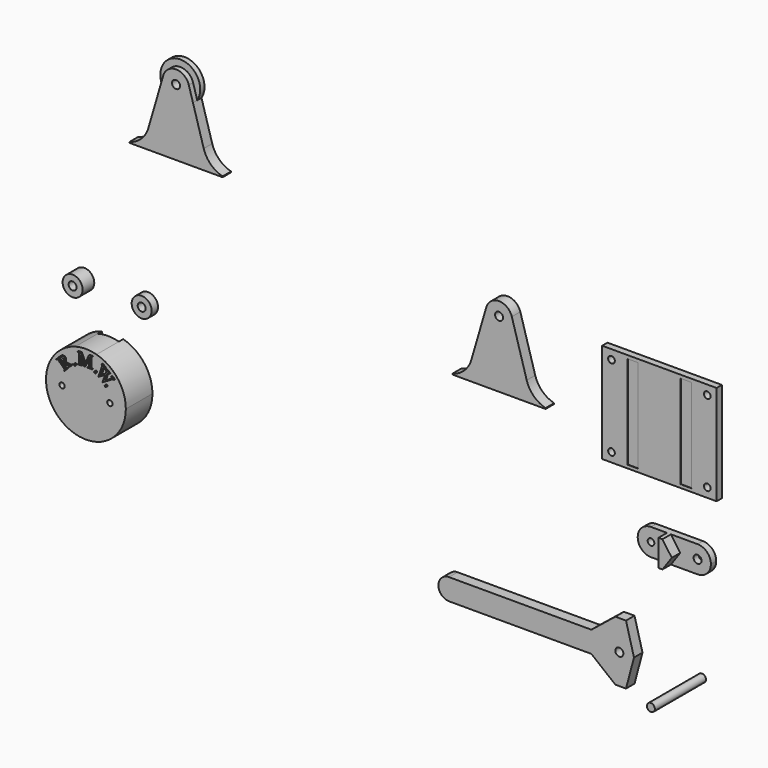
from build123d import *

# Parameters (mm, degrees)
F0_R      = 3
F1_DEPTH  = 8
F2_R      = 3
F3_DEPTH  = 8
F4_R      = 3
F5_DEPTH  = 48
F7_DEPTH  = 21
F6_R      = 2
F8_DEPTH  = 25
F9_DEPTH  = 1
F10_R     = 7.5
F10_R_2   = 3
F12_DEPTH = 6
F11_R     = 7.5
F11_R_2   = 3
F13_DEPTH = 11
F16_DEPTH = 4
F15_R     = 3
F17_DEPTH = 8
F14_W     = 86
F14_H     = 75
F14_R     = 2.5
F14_W_2   = 8
F14_H_2   = 70.1
F18_DEPTH = 5
F19_DEPTH = 4.7
F20_R     = 2.5
F21_DEPTH = 5
F20_R_2   = 7.5
F22_START = 0.2
F20_R_3   = 3
F22_DEPTH = 4.8
F23_DEPTH = 13


# Not quite as in the source:
# - ends of sketch curves that miss each other by under 0.0002 mm in the source are joined


with BuildPart() as f1:
    # F0 (on Front) → F1 (new body)
    with BuildSketch(Plane.XZ):
        with BuildLine():
            Line((91.7526111007, 74.1948067945), (91.7526111007, 73.5597237945))
            Line((91.7526111007, 73.5597237945), (161.7526111007, 73.5597237945))
            Line((161.7526111007, 73.5597237945), (161.7526111007, 74.1948067945))
            ThreePointArc((161.7526111007, 74.1948067945), (152.8321860899, 79.1993001406), (147.5526111007, 87.9597237945))
            Line((147.5526111007, 87.9597237945), (136.3526111007, 126.3597237945))
            ThreePointArc((136.3526111007, 126.3597237945), (126.7526111007, 133.5597237945), (117.1526111007, 126.3597237945))
            Line((117.1526111007, 126.3597237945), (105.9526111007, 87.9597237945))
            ThreePointArc((105.9526111007, 87.9597237945), (100.6730361115, 79.1993001406), (91.7526111007, 74.1948067945))
        make_face()
        with Locations((126.7526111007, 123.5597237945)):
            Circle(F0_R, mode=Mode.SUBTRACT)
    extrude(amount=F1_DEPTH)


with BuildPart() as f3:
    # F2 (on Front) → F3 (new body)
    with BuildSketch(Plane.XZ):
        with BuildLine():
            Line((228.1742408276, -69.2982090712), (222.1742408276, -46.7982090712))
            Line((222.1742408276, -46.7982090712), (214.1742408276, -46.7982090712))
            Line((214.1742408276, -46.7982090712), (196.1742408276, -61.2982090712))
            Line((196.1742408276, -61.2982090712), (89.1742408276, -61.2982090712))
            ThreePointArc((89.1742408276, -61.2982090712), (83.5173865781, -63.6413548217), (81.1742408276, -69.2982090712))
            ThreePointArc((81.1742408276, -69.2982090712), (83.5173865781, -74.9550633207), (89.1742408276, -77.2982090712))
            Line((89.1742408276, -77.2982090712), (196.1742408276, -77.2982090712))
            Line((196.1742408276, -77.2982090712), (214.1742408276, -91.7982090712))
            Line((214.1742408276, -91.7982090712), (222.1742408276, -91.7982090712))
            Line((222.1742408276, -91.7982090712), (228.1742408276, -69.2982090712))
        make_face()
        with Locations((217.1742408276, -69.2982090712)):
            Circle(F2_R, mode=Mode.SUBTRACT)
    extrude(amount=F3_DEPTH)


with BuildPart() as f5:
    # F4 (on Front) → F5 (new body)
    with BuildSketch(Plane.XZ):
        with Locations((272.8815972805, -71.5365037322)):
            Circle(F4_R)
    extrude(amount=F5_DEPTH)


with BuildPart() as f7:
    # F6 (on Front) → F7 (new body)
    with BuildSketch(Plane.XZ):
        with BuildLine():
            Line((-198.1619641029, -16.3318043726), (-198.0776991029, -16.2824186042))
            Line((-198.0776991029, -16.2824186042), (-197.9450911029, -16.2339666042))
            Line((-197.9450911029, -16.2339666042), (-197.8122691029, -16.2133986042))
            Line((-197.8122691029, -16.2133986042), (-197.6792331029, -16.2207146042))
            Line((-197.6792331029, -16.2207146042), (-197.5459821029, -16.2559146042))
            Line((-197.5459821029, -16.2559146042), (-197.4216611029, -16.3151236042))
            Line((-197.4216611029, -16.3151236042), (-197.3154121029, -16.3944676042))
            Line((-197.3154121029, -16.3944676042), (-197.2272371029, -16.4939466042))
            Line((-197.2272371029, -16.4939466042), (-197.1571341029, -16.6135606042))
            Line((-197.1571341029, -16.6135606042), (-197.1097611029, -16.7438786042))
            Line((-197.1097611029, -16.7438786042), (-197.0897731029, -16.8754666042))
            Line((-197.0897731029, -16.8754666042), (-197.0971721029, -17.0083266042))
            Line((-197.0971721029, -17.0083266042), (-197.1319571029, -17.1424586042))
            Line((-197.1319571029, -17.1424586042), (-197.1905861029, -17.2680136042))
            Line((-197.1905861029, -17.2680136042), (-197.2695151029, -17.3751426042))
            Line((-197.2695151029, -17.3751426042), (-197.3687451029, -17.4638476042))
            Line((-197.3687451029, -17.4638476042), (-197.4882761029, -17.5341266042))
            Line((-197.4882761029, -17.5341266042), (-197.6185941029, -17.5814996042))
            Line((-197.6185941029, -17.5814996042), (-197.7501821029, -17.6014866042))
            Line((-197.7501821029, -17.6014866042), (-197.8830431029, -17.5940876042))
            Line((-197.8830431029, -17.5940876042), (-198.0171741029, -17.5593026042))
            Line((-198.0171741029, -17.5593026042), (-198.1427291029, -17.5006746042))
            Line((-198.1427291029, -17.5006746042), (-198.1619641029, -17.4865028638))
            Line((-198.1619641029, -17.4865028638), (-198.1619641029, -63.2965836042))
            ThreePointArc((-198.1619641029, -63.2965836042), (-190.1619641029, -64.3829186042), (-182.1619642084, -63.296583223))
            Line((-182.1619642084, -63.296583223), (-182.1619641029, -17.5489829879))
            Line((-182.1619641029, -17.5489829879), (-182.2444761029, -17.5865666042))
            Line((-182.2444761029, -17.5865666042), (-182.3789311029, -17.6200826042))
            Line((-182.3789311029, -17.6200826042), (-182.5118551029, -17.6262246042))
            Line((-182.5118551029, -17.6262246042), (-182.6432491029, -17.6049946042))
            Line((-182.6432491029, -17.6049946042), (-182.7731131029, -17.5563916042))
            Line((-182.7731131029, -17.5563916042), (-182.8919741029, -17.4849856042))
            Line((-182.8919741029, -17.4849856042), (-182.9903611029, -17.3953476042))
            Line((-182.9903611029, -17.3953476042), (-183.0682741029, -17.2874766042))
            Line((-183.0682741029, -17.2874766042), (-183.1257131029, -17.1613736042))
            Line((-183.1257131029, -17.1613736042), (-183.1592291029, -17.0269186042))
            Line((-183.1592291029, -17.0269186042), (-183.1653711029, -16.8939946042))
            Line((-183.1653711029, -16.8939946042), (-183.1441411029, -16.7626006042))
            Line((-183.1441411029, -16.7626006042), (-183.0955381029, -16.6327366042))
            Line((-183.0955381029, -16.6327366042), (-183.0230321029, -16.5115956042))
            Line((-183.0230321029, -16.5115956042), (-182.9328011029, -16.4119806042))
            Line((-182.9328011029, -16.4119806042), (-182.8248461029, -16.3338916042))
            Line((-182.8248461029, -16.3338916042), (-182.6991651029, -16.2773296042))
            Line((-182.6991651029, -16.2773296042), (-182.5653031029, -16.2450426042))
            Line((-182.5653031029, -16.2450426042), (-182.4328021029, -16.2397766042))
            Line((-182.4328021029, -16.2397766042), (-182.3016621029, -16.2615336042))
            Line((-182.3016621029, -16.2615336042), (-182.1718831029, -16.3103116042))
            Line((-182.1718831029, -16.3103116042), (-182.1619641029, -16.3162483805))
            Line((-182.1619641029, -16.3162483805), (-182.1619641029, -5.4692546042))
            ThreePointArc((-182.1619641029, -5.4692546042), (-190.1619641029, -4.3829186042), (-198.1619642544, -5.4692540565))
            Line((-198.1619642544, -5.4692540565), (-198.1619641029, -16.3318043726))
        make_face()
        Polygon((-190.3483751029, -15.8450716042), (-190.5540121029, -15.8482386042), (-193.9287881029, -8.7884576042), (-193.8418381029, -14.4341396042), (-193.8258881029, -14.7868326042), (-193.7900351029, -15.0659826042), (-193.7646451029, -15.1779796042), (-193.7342781029, -15.2715896042), (-193.6989361029, -15.3468136042), (-193.6586181029, -15.4036526042), (-193.5958461029, -15.4640416042), (-193.5248261029, -15.5161226042), (-193.4455591029, -15.5598956042), (-193.3580441029, -15.5953606042), (-193.2622811029, -15.6225186042), (-193.1582721029, -15.6413676042), (-193.0460141029, -15.6519106042), (-192.9255091029, -15.6541446042), (-192.6264001029, -15.6495376042), (-192.6228491029, -15.8801016042), (-195.5640881029, -15.9253996042), (-195.5676391029, -15.6948366042), (-195.2685301029, -15.6902296042), (-195.1395001029, -15.6831786042), (-195.0203631029, -15.6661506042), (-194.9111181029, -15.6391466042), (-194.8117671029, -15.6021666042), (-194.7223071029, -15.5552106042), (-194.6427401029, -15.4982786042), (-194.5730661029, -15.4313706042), (-194.5132851029, -15.3544866042), (-194.4820451029, -15.2961556042), (-194.4553351029, -15.2219236042), (-194.4331541029, -15.1317886042), (-194.4155041029, -15.0257526042), (-194.3937951029, -14.7659726042), (-194.3902051029, -14.4425856042), (-194.4752351029, -8.9215316042), (-194.4870431029, -8.6607096042), (-194.5138301029, -8.4390746042), (-194.5555951029, -8.2566266042), (-194.6123401029, -8.1133636042), (-194.6664471029, -8.0275206042), (-194.7387451029, -7.9493596042), (-194.8292331029, -7.8788796042), (-194.9379131029, -7.8160816042), (-195.0732921029, -7.7649926042), (-195.2438781029, -7.7296376042), (-195.4496721029, -7.7100176042), (-195.6906731029, -7.7061336042), (-195.6942241029, -7.4755696042), (-193.3013521029, -7.4387176042), (-190.1336601029, -14.0030546042), (-187.2194691029, -7.3450506042), (-184.8265971029, -7.3081976042), (-184.8230461029, -7.5387606042), (-185.1159231029, -7.5432716042), (-185.2464131029, -7.5503456042), (-185.3668161029, -7.5673926042), (-185.4771321029, -7.5944126042), (-185.5773601029, -7.6314056042), (-185.6675011029, -7.6783726042), (-185.7475541029, -7.7353116042), (-185.8175211029, -7.8022246042), (-185.8774001029, -7.8791106042), (-185.9086401029, -7.9374406042), (-185.9353501029, -8.0116736042), (-185.9575301029, -8.1018076042), (-185.9751801029, -8.2078446042), (-185.9968901029, -8.4676236042), (-186.0004801029, -8.7910116042), (-185.9154501029, -14.3120656042), (-185.8991101029, -14.6647526042), (-185.8831851029, -14.8135126042), (-185.8620891029, -14.9438846042), (-185.8358221029, -15.0558676042), (-185.8043851029, -15.1494606042), (-185.7677771029, -15.2246656042), (-185.7259981029, -15.2814826042), (-185.6632261029, -15.3418706042), (-185.5922061029, -15.3939516042), (-185.5129391029, -15.4377246042), (-185.4254241029, -15.4731896042), (-185.3296621029, -15.5003476042), (-185.2256521029, -15.5191976042), (-185.1133941029, -15.5297396042), (-184.9928891029, -15.5319746042), (-184.7000121029, -15.5274636042), (-184.6964611029, -15.7580266042), (-188.2857691029, -15.8133056042), (-188.2893201029, -15.5827426042), (-187.9902111029, -15.5781356042), (-187.8598181029, -15.5710636042), (-187.7397071029, -15.5540206042), (-187.6298781029, -15.5270086042), (-187.5303321029, -15.4900256042), (-187.4410671029, -15.4430726042), (-187.3620851029, -15.3861496042), (-187.2933841029, -15.3192566042), (-187.2349661029, -15.2423926042), (-187.2037261029, -15.1840626042), (-187.1770151029, -15.1098296042), (-187.1548351029, -15.0196956042), (-187.1371851029, -14.9136586042), (-187.1154761029, -14.6538796042), (-187.1118861029, -14.3304916042), (-187.1988351029, -8.6848096042), align=None, mode=Mode.SUBTRACT)
        Polygon((-193.9287881029, -8.7884576042), (-190.5540121029, -15.8482386042), (-190.3483751029, -15.8450716042), (-187.1988351029, -8.6848096042), (-187.1118861029, -14.3304916042), (-187.1154761029, -14.6538796042), (-187.1371851029, -14.9136586042), (-187.1548351029, -15.0196956042), (-187.1770151029, -15.1098296042), (-187.2037261029, -15.1840626042), (-187.2349661029, -15.2423926042), (-187.2933841029, -15.3192566042), (-187.3620851029, -15.3861496042), (-187.4410671029, -15.4430726042), (-187.5303321029, -15.4900256042), (-187.6298781029, -15.5270086042), (-187.7397071029, -15.5540206042), (-187.8598181029, -15.5710636042), (-187.9902111029, -15.5781356042), (-188.2893201029, -15.5827426042), (-188.2857691029, -15.8133056042), (-184.6964611029, -15.7580266042), (-184.7000121029, -15.5274636042), (-184.9928891029, -15.5319746042), (-185.1133941029, -15.5297396042), (-185.2256521029, -15.5191976042), (-185.3296621029, -15.5003476042), (-185.4254241029, -15.4731896042), (-185.5129391029, -15.4377246042), (-185.5922061029, -15.3939516042), (-185.6632261029, -15.3418706042), (-185.7259981029, -15.2814826042), (-185.7677771029, -15.2246656042), (-185.8043851029, -15.1494606042), (-185.8358221029, -15.0558676042), (-185.8620891029, -14.9438846042), (-185.8831851029, -14.8135126042), (-185.8991101029, -14.6647526042), (-185.9154501029, -14.3120656042), (-186.0004801029, -8.7910116042), (-185.9968901029, -8.4676236042), (-185.9751801029, -8.2078446042), (-185.9575301029, -8.1018076042), (-185.9353501029, -8.0116736042), (-185.9086401029, -7.9374406042), (-185.8774001029, -7.8791106042), (-185.8175211029, -7.8022246042), (-185.7475541029, -7.7353116042), (-185.6675011029, -7.6783726042), (-185.5773601029, -7.6314056042), (-185.4771321029, -7.5944126042), (-185.3668161029, -7.5673926042), (-185.2464131029, -7.5503456042), (-185.1159231029, -7.5432716042), (-184.8230461029, -7.5387606042), (-184.8265971029, -7.3081976042), (-187.2194691029, -7.3450506042), (-190.1336601029, -14.0030546042), (-193.3013521029, -7.4387176042), (-195.6942241029, -7.4755696042), (-195.6906731029, -7.7061336042), (-195.4496721029, -7.7100176042), (-195.2438781029, -7.7296376042), (-195.0732921029, -7.7649926042), (-194.9379131029, -7.8160816042), (-194.8292331029, -7.8788796042), (-194.7387451029, -7.9493596042), (-194.6664471029, -8.0275206042), (-194.6123401029, -8.1133636042), (-194.5555951029, -8.2566266042), (-194.5138301029, -8.4390746042), (-194.4870431029, -8.6607096042), (-194.4752351029, -8.9215316042), (-194.3902051029, -14.4425856042), (-194.3937951029, -14.7659726042), (-194.4155041029, -15.0257526042), (-194.4331541029, -15.1317886042), (-194.4553351029, -15.2219236042), (-194.4820451029, -15.2961556042), (-194.5132851029, -15.3544866042), (-194.5730661029, -15.4313706042), (-194.6427401029, -15.4982786042), (-194.7223071029, -15.5552106042), (-194.8117671029, -15.6021666042), (-194.9111181029, -15.6391466042), (-195.0203631029, -15.6661506042), (-195.1395001029, -15.6831786042), (-195.2685301029, -15.6902296042), (-195.5676391029, -15.6948366042), (-195.5640881029, -15.9253996042), (-192.6228491029, -15.8801016042), (-192.6264001029, -15.6495376042), (-192.9255091029, -15.6541446042), (-193.0460141029, -15.6519106042), (-193.1582721029, -15.6413676042), (-193.2622811029, -15.6225186042), (-193.3580441029, -15.5953606042), (-193.4455591029, -15.5598956042), (-193.5248261029, -15.5161226042), (-193.5958461029, -15.4640416042), (-193.6586181029, -15.4036526042), (-193.6989361029, -15.3468136042), (-193.7342781029, -15.2715896042), (-193.7646451029, -15.1779796042), (-193.7900351029, -15.0659826042), (-193.8258881029, -14.7868326042), (-193.8418381029, -14.4341396042), align=None)
        Polygon((-182.1619641029, -17.5489829879), (-182.1619641029, -16.3162483805), (-182.1718831029, -16.3103116042), (-182.3016621029, -16.2615336042), (-182.4328021029, -16.2397766042), (-182.5653031029, -16.2450426042), (-182.6991651029, -16.2773296042), (-182.8248461029, -16.3338916042), (-182.9328011029, -16.4119806042), (-183.0230321029, -16.5115956042), (-183.0955381029, -16.6327366042), (-183.1441411029, -16.7626006042), (-183.1653711029, -16.8939946042), (-183.1592291029, -17.0269186042), (-183.1257131029, -17.1613736042), (-183.0682741029, -17.2874766042), (-182.9903611029, -17.3953476042), (-182.8919741029, -17.4849856042), (-182.7731131029, -17.5563916042), (-182.6432491029, -17.6049946042), (-182.5118551029, -17.6262246042), (-182.3789311029, -17.6200826042), (-182.2444761029, -17.5865666042), align=None)
        Polygon((-197.9450911029, -16.2339666042), (-198.0776991029, -16.2824186042), (-198.1619641029, -16.3318043726), (-198.1619641029, -17.4865028638), (-198.1427291029, -17.5006746042), (-198.0171741029, -17.5593026042), (-197.8830431029, -17.5940876042), (-197.7501821029, -17.6014866042), (-197.6185941029, -17.5814996042), (-197.4882761029, -17.5341266042), (-197.3687451029, -17.4638476042), (-197.2695151029, -17.3751426042), (-197.1905861029, -17.2680136042), (-197.1319571029, -17.1424586042), (-197.0971721029, -17.0083266042), (-197.0897731029, -16.8754666042), (-197.1097611029, -16.7438786042), (-197.1571341029, -16.6135606042), (-197.2272371029, -16.4939466042), (-197.3154121029, -16.3944676042), (-197.4216611029, -16.3151236042), (-197.5459821029, -16.2559146042), (-197.6792331029, -16.2207146042), (-197.8122691029, -16.2133986042), align=None)
    extrude(amount=-F7_DEPTH)

    # F6 (on Front) → F8 (join)
    with BuildSketch(Plane.XZ):
        with BuildLine():
            Line((-198.1973131029, -16.3525216042), (-198.1619641029, -16.3318043726))
            Line((-198.1619641029, -16.3318043726), (-198.1619641029, -5.4692546042))
            ThreePointArc((-198.1619641029, -5.4692546042), (-220.1619641029, -34.3829187375), (-198.1619639974, -63.296583223))
            Line((-198.1619639974, -63.296583223), (-198.1619641029, -17.4865028638))
            Line((-198.1619641029, -17.4865028638), (-198.2498591029, -17.4217446042))
            Line((-198.2498591029, -17.4217446042), (-198.3385631029, -17.3225146042))
            Line((-198.3385631029, -17.3225146042), (-198.4088421029, -17.2029836042))
            Line((-198.4088421029, -17.2029836042), (-198.4572941029, -17.0703756042))
            Line((-198.4572941029, -17.0703756042), (-198.4778621029, -16.9375536042))
            Line((-198.4778621029, -16.9375536042), (-198.4705461029, -16.8045176042))
            Line((-198.4705461029, -16.8045176042), (-198.4353461029, -16.6712666042))
            Line((-198.4353461029, -16.6712666042), (-198.3761371029, -16.5469456042))
            Line((-198.3761371029, -16.5469456042), (-198.2967921029, -16.4406966042))
            Line((-198.2967921029, -16.4406966042), (-198.1973131029, -16.3525216042))
        make_face()
        with Locations((-208.1619641029, -34.3829186042)):
            Circle(F6_R, mode=Mode.SUBTRACT)
        Polygon((-200.0576071029, -17.6949796042), (-199.8936781029, -17.8571486042), (-201.4803091029, -19.4610036042), (-206.3010501029, -18.7158246042), (-206.6559751029, -19.0923246042), (-206.7809131029, -19.2141886042), (-206.9234311029, -19.3449606042), (-205.1777981029, -21.0718476042), (-204.9134341029, -21.3180316042), (-204.7956441029, -21.4153806042), (-204.6874491029, -21.4955656042), (-204.5888491029, -21.5585886042), (-204.4998441029, -21.6044496042), (-204.4204351029, -21.6331476042), (-204.3506201029, -21.6446836042), (-204.2606891029, -21.6451616042), (-204.1716461029, -21.6343526042), (-204.0834901029, -21.6122556042), (-203.9962211029, -21.5788706042), (-203.9098401029, -21.5341976042), (-203.8243451029, -21.4782366042), (-203.7397381029, -21.4109886042), (-203.6560181029, -21.3324516042), (-203.4237211029, -21.0976336042), (-203.2597921029, -21.2598026042), (-205.8062921029, -23.8339466042), (-205.9702221029, -23.6717766042), (-205.7466911029, -23.4458196042), (-205.6596901029, -23.3501196042), (-205.5871531029, -23.2535346042), (-205.5290821029, -23.1560626042), (-205.4854751029, -23.0577056042), (-205.4563331029, -22.9584626042), (-205.4416561029, -22.8583326042), (-205.4414441029, -22.7573176042), (-205.4556971029, -22.6554166042), (-205.4743451029, -22.5938216042), (-205.5076391029, -22.5234906042), (-205.6181611029, -22.3566266042), (-205.7872621029, -22.1548226042), (-206.0149441029, -21.9180806042), (-209.8960961029, -18.0786066042), (-210.1604611029, -17.8324226042), (-210.2782511029, -17.7350736042), (-210.3864451029, -17.6548886042), (-210.4850451029, -17.5918646042), (-210.5740501029, -17.5460046042), (-210.6534601029, -17.5173066042), (-210.7232751029, -17.5057706042), (-210.8143011029, -17.5064006042), (-210.9044401029, -17.5183166042), (-210.9936921029, -17.5415216042), (-211.0820561029, -17.5760146042), (-211.1695331029, -17.6217946042), (-211.2561241029, -17.6788636042), (-211.3418261029, -17.7472196042), (-211.4266421029, -17.8268636042), (-211.6501731029, -18.0528206042), (-211.8141031029, -17.8906516042), (-209.6489201029, -15.7019646042), (-209.1979291029, -15.2635246042), (-208.9892111029, -15.0743486042), (-208.7916771029, -14.9052006042), (-208.6053271029, -14.7560826042), (-208.4301621029, -14.6269926042), (-208.2661811029, -14.5179326042), (-208.1133851029, -14.4289016042), (-207.9646351029, -14.3556606042), (-207.8127931029, -14.2939706042), (-207.6578591029, -14.2438326042), (-207.4998331029, -14.2052456042), (-207.3387151029, -14.1782096042), (-207.1745041029, -14.1627256042), (-207.0072021029, -14.1587926042), (-206.8368071029, -14.1664106042), (-206.6675141029, -14.1869806042), (-206.5035131029, -14.2219016042), (-206.3448061029, -14.2711726042), (-206.1913921029, -14.3347956042), (-206.0432721029, -14.4127686042), (-205.9004451029, -14.5050926042), (-205.7629121029, -14.6117676042), (-205.6306721029, -14.7327946042), (-205.5000841029, -14.8731436042), (-205.3852271029, -15.0202576042), (-205.2861021029, -15.1741356042), (-205.2027091029, -15.3347766042), (-205.1350481029, -15.5021826042), (-205.0831191029, -15.6763536042), (-205.0469221029, -15.8572876042), (-205.0264561029, -16.0449856042), (-205.0237241029, -16.2385636042), (-205.0407281029, -16.4371366042), (-205.0774661029, -16.6407056042), (-205.1339391029, -16.8492706042), (-205.2101481029, -17.0628296042), (-205.3060911029, -17.2813856042), (-205.4217701029, -17.5049356042), (-205.5571841029, -17.7334816042), (-202.6064751029, -18.1979026042), (-202.1315651029, -18.2617176042), (-201.7212911029, -18.2911766042), (-201.5403921029, -18.2930236042), (-201.3756531029, -18.2862816042), (-201.2270721029, -18.2709506042), (-201.0946511029, -18.2470306042), (-200.9696481029, -18.2137176042), (-200.8433221029, -18.1702056042), (-200.7156751029, -18.1164966042), (-200.5867061029, -18.0525896042), (-200.4564141029, -17.9784836042), (-200.3248011029, -17.8941806042), align=None, mode=Mode.SUBTRACT)
        with BuildLine():
            ThreePointArc((-160.1619641029, -34.3829186042), (-166.2872912827, -16.2170165422), (-182.1619639514, -5.4692540565))
            Line((-182.1619639514, -5.4692540565), (-182.1619641029, -16.3162483805))
            Line((-182.1619641029, -16.3162483805), (-182.0507421029, -16.3828176042))
            Line((-182.0507421029, -16.3828176042), (-181.9511271029, -16.4730486042))
            Line((-181.9511271029, -16.4730486042), (-181.8730381029, -16.5810036042))
            Line((-181.8730381029, -16.5810036042), (-181.8164761029, -16.7066846042))
            Line((-181.8164761029, -16.7066846042), (-181.7841891029, -16.8405466042))
            Line((-181.7841891029, -16.8405466042), (-181.7789231029, -16.9730476042))
            Line((-181.7789231029, -16.9730476042), (-181.8006801029, -17.1041876042))
            Line((-181.8006801029, -17.1041876042), (-181.8494581029, -17.2339666042))
            Line((-181.8494581029, -17.2339666042), (-181.9208641029, -17.3528276042))
            Line((-181.9208641029, -17.3528276042), (-182.0105021029, -17.4512146042))
            Line((-182.0105021029, -17.4512146042), (-182.1183731029, -17.5291276042))
            Line((-182.1183731029, -17.5291276042), (-182.1619641029, -17.5489829879))
            Line((-182.1619641029, -17.5489829879), (-182.1619641029, -63.2965836042))
            ThreePointArc((-182.1619641029, -63.2965836042), (-166.2872913634, -52.5488207723), (-160.1619641029, -34.3829186042))
        make_face()
        with Locations((-172.1619641029, -34.3829186042)):
            Circle(F6_R, mode=Mode.SUBTRACT)
        Polygon((-174.0892951029, -22.9184336042), (-173.9963871029, -23.0213406042), (-173.9220431029, -23.1413636042), (-173.8749611029, -23.2672526042), (-173.8551391029, -23.3990076042), (-173.8625781029, -23.5366276042), (-173.8953381029, -23.6703746042), (-173.9514811029, -23.7905096042), (-174.0310061029, -23.8970306042), (-174.1339141029, -23.9899386042), (-174.2519131029, -24.0627616042), (-174.3767111029, -24.1090246042), (-174.5083101029, -24.1287296042), (-174.6467101029, -24.1218756042), (-174.7815471029, -24.0899346042), (-174.9024591029, -24.0343766042), (-175.0094481029, -23.9552016042), (-175.1025121029, -23.8524116042), (-175.1753341029, -23.7344126042), (-175.2215981029, -23.6096146042), (-175.2413031029, -23.4780156042), (-175.2344491029, -23.3396156042), (-175.2025071029, -23.2047786042), (-175.1469491029, -23.0838656042), (-175.0677751029, -22.9768776042), (-174.9649851029, -22.8838136042), (-174.8449621029, -22.8094706042), (-174.7190731029, -22.7623876042), (-174.5873181029, -22.7425656042), (-174.4496981029, -22.7500046042), (-174.3159501029, -22.7827656042), (-174.1958161029, -22.8389086042), align=None, mode=Mode.SUBTRACT)
        Polygon((-170.2892841029, -15.7694166042), (-168.3366211029, -17.3687426042), (-168.4827321029, -17.5471346042), (-168.6091621029, -17.4531486042), (-168.7329161029, -17.3804856042), (-168.8539961029, -17.3291466042), (-168.9724021029, -17.2991306042), (-169.0967101029, -17.2904606042), (-169.2355011029, -17.3031596042), (-169.3887721029, -17.3372276042), (-169.5565251029, -17.3926656042), (-169.7047171029, -17.4611036042), (-169.9146511029, -17.5766476042), (-170.1863281029, -17.7392976042), (-170.5197481029, -17.9490536042), (-176.6584381029, -21.7261286042), (-176.8512931029, -21.5681706042), (-174.9173611029, -16.1677986042), (-179.8212701029, -19.1356156042), (-179.9948401029, -18.9934526042), (-177.4913391029, -11.9731406042), (-177.2726431029, -11.3446726042), (-177.1777641029, -11.0296636042), (-177.1601301029, -10.9008646042), (-177.1608611029, -10.7766606042), (-177.1799551029, -10.6570516042), (-177.2174141029, -10.5420366042), (-177.2760041029, -10.4288476042), (-177.3584911029, -10.3147136042), (-177.4648761029, -10.1996356042), (-177.5951591029, -10.0836136042), (-177.4490471029, -9.9052226042), (-175.0287101029, -11.8875966042), (-175.1748211029, -12.0659886042), (-175.2905341029, -11.9712136042), (-175.4166911029, -11.8799686042), (-175.5396281029, -11.8155276042), (-175.6593451029, -11.7778926042), (-175.7758421029, -11.7670616042), (-175.8847591029, -11.7795566042), (-175.9817381029, -11.8119006042), (-176.0667781029, -11.8640916042), (-176.1398801029, -11.9361316042), (-176.2181871029, -12.0587866042), (-176.3148971029, -12.2580056042), (-176.4300081029, -12.5337856042), (-176.5635201029, -12.8861286042), (-178.2813621029, -17.6095766042), (-174.6415771029, -15.3786516042), (-174.3842521029, -14.6710556042), (-174.1791821029, -14.1059426042), (-174.1355511029, -13.9463256042), (-174.1008571029, -13.7914736042), (-174.0751001029, -13.6413846042), (-174.0582791029, -13.4960596042), (-174.0590831029, -13.3544256042), (-174.0861971029, -13.2154086042), (-174.1455231029, -13.0419536042), (-174.2245941029, -12.8926046042), (-174.2666611029, -12.8370036042), (-174.3249481029, -12.7741596042), (-174.4901841029, -12.6267396042), (-174.3440721029, -12.4483476042), (-171.7983791029, -14.5333946042), (-171.9444901029, -14.7117866042), (-172.1180601029, -14.5696236042), (-172.2499421029, -14.4736896042), (-172.3755911029, -14.4070286042), (-172.4950071029, -14.3696396042), (-172.6081891029, -14.3615236042), (-172.7146151029, -14.3795836042), (-172.8137641029, -14.4207226042), (-172.9056341029, -14.4849416042), (-172.9902271029, -14.5722406042), (-173.0961221029, -14.7291946042), (-173.2124131029, -14.9541636042), (-173.3390981029, -15.2471496042), (-173.4761781029, -15.6081506042), (-175.1329941029, -20.1882426042), (-170.9392081029, -17.6054946042), (-170.6203191029, -17.4054876042), (-170.3654631029, -17.2295636042), (-170.1746391029, -17.0777246042), (-170.0478471029, -16.9499696042), (-170.0075441029, -16.8918486042), (-169.9774611029, -16.8283786042), (-169.9575971029, -16.7595586042), (-169.9479531029, -16.6853896042), (-169.9486401029, -16.6103106042), (-169.9597711029, -16.5387626042), (-169.9813451029, -16.4707436042), (-170.0133631029, -16.4062546042), (-170.0877131029, -16.2960166042), (-170.1828341029, -16.1828626042), (-170.2987291029, -16.0667936042), (-170.4353951029, -15.9478086042), align=None, mode=Mode.SUBTRACT)
        Polygon((-201.4803091029, -19.4610036042), (-199.8936781029, -17.8571486042), (-200.0576071029, -17.6949796042), (-200.3248011029, -17.8941806042), (-200.4564141029, -17.9784836042), (-200.5867061029, -18.0525896042), (-200.7156751029, -18.1164966042), (-200.8433221029, -18.1702056042), (-200.9696481029, -18.2137176042), (-201.0946511029, -18.2470306042), (-201.2270721029, -18.2709506042), (-201.3756531029, -18.2862816042), (-201.5403921029, -18.2930236042), (-201.7212911029, -18.2911766042), (-202.1315651029, -18.2617176042), (-202.6064751029, -18.1979026042), (-205.5571841029, -17.7334816042), (-205.4217701029, -17.5049356042), (-205.3060911029, -17.2813856042), (-205.2101481029, -17.0628296042), (-205.1339391029, -16.8492706042), (-205.0774661029, -16.6407056042), (-205.0407281029, -16.4371366042), (-205.0237241029, -16.2385636042), (-205.0264561029, -16.0449856042), (-205.0469221029, -15.8572876042), (-205.0831191029, -15.6763536042), (-205.1350481029, -15.5021826042), (-205.2027091029, -15.3347766042), (-205.2861021029, -15.1741356042), (-205.3852271029, -15.0202576042), (-205.5000841029, -14.8731436042), (-205.6306721029, -14.7327946042), (-205.7629121029, -14.6117676042), (-205.9004451029, -14.5050926042), (-206.0432721029, -14.4127686042), (-206.1913921029, -14.3347956042), (-206.3448061029, -14.2711726042), (-206.5035131029, -14.2219016042), (-206.6675141029, -14.1869806042), (-206.8368071029, -14.1664106042), (-207.0072021029, -14.1587926042), (-207.1745041029, -14.1627256042), (-207.3387151029, -14.1782096042), (-207.4998331029, -14.2052456042), (-207.6578591029, -14.2438326042), (-207.8127931029, -14.2939706042), (-207.9646351029, -14.3556606042), (-208.1133851029, -14.4289016042), (-208.2661811029, -14.5179326042), (-208.4301621029, -14.6269926042), (-208.6053271029, -14.7560826042), (-208.7916771029, -14.9052006042), (-208.9892111029, -15.0743486042), (-209.1979291029, -15.2635246042), (-209.6489201029, -15.7019646042), (-211.8141031029, -17.8906516042), (-211.6501731029, -18.0528206042), (-211.4266421029, -17.8268636042), (-211.3418261029, -17.7472196042), (-211.2561241029, -17.6788636042), (-211.1695331029, -17.6217946042), (-211.0820561029, -17.5760146042), (-210.9936921029, -17.5415216042), (-210.9044401029, -17.5183166042), (-210.8143011029, -17.5064006042), (-210.7232751029, -17.5057706042), (-210.6534601029, -17.5173066042), (-210.5740501029, -17.5460046042), (-210.4850451029, -17.5918646042), (-210.3864451029, -17.6548886042), (-210.2782511029, -17.7350736042), (-210.1604611029, -17.8324226042), (-209.8960961029, -18.0786066042), (-206.0149441029, -21.9180806042), (-205.7872621029, -22.1548226042), (-205.6181611029, -22.3566266042), (-205.5076391029, -22.5234906042), (-205.4743451029, -22.5938216042), (-205.4556971029, -22.6554166042), (-205.4414441029, -22.7573176042), (-205.4416561029, -22.8583326042), (-205.4563331029, -22.9584626042), (-205.4854751029, -23.0577056042), (-205.5290821029, -23.1560626042), (-205.5871531029, -23.2535346042), (-205.6596901029, -23.3501196042), (-205.7466911029, -23.4458196042), (-205.9702221029, -23.6717766042), (-205.8062921029, -23.8339466042), (-203.2597921029, -21.2598026042), (-203.4237211029, -21.0976336042), (-203.6560181029, -21.3324516042), (-203.7397381029, -21.4109886042), (-203.8243451029, -21.4782366042), (-203.9098401029, -21.5341976042), (-203.9962211029, -21.5788706042), (-204.0834901029, -21.6122556042), (-204.1716461029, -21.6343526042), (-204.2606891029, -21.6451616042), (-204.3506201029, -21.6446836042), (-204.4204351029, -21.6331476042), (-204.4998441029, -21.6044496042), (-204.5888491029, -21.5585886042), (-204.6874491029, -21.4955656042), (-204.7956441029, -21.4153806042), (-204.9134341029, -21.3180316042), (-205.1777981029, -21.0718476042), (-206.9234311029, -19.3449606042), (-206.7809131029, -19.2141886042), (-206.6559751029, -19.0923246042), (-206.3010501029, -18.7158246042), align=None)
        Polygon((-207.0557021029, -18.9248176042), (-207.2025551029, -19.0688346042), (-209.7013791029, -16.5968446042), (-209.5324821029, -16.3524526042), (-209.3755261029, -16.1411766042), (-209.2305101029, -15.9630176042), (-209.0974341029, -15.8179736042), (-208.9519161029, -15.6818826042), (-208.8024441029, -15.5638116042), (-208.6490181029, -15.4637596042), (-208.4916401029, -15.3817276042), (-208.3303081029, -15.3177146042), (-208.1650231029, -15.2717206042), (-207.9957851029, -15.2437456042), (-207.8225931029, -15.2337906042), (-207.6495811029, -15.2416016042), (-207.4808811029, -15.2669256042), (-207.3164941029, -15.3097626042), (-207.1564181029, -15.3701126042), (-207.0006561029, -15.4479756042), (-206.8492051029, -15.5433516042), (-206.7020671029, -15.6562416042), (-206.5592411029, -15.7866436042), (-206.4251791029, -15.9327586042), (-206.3109771029, -16.0862106042), (-206.2166351029, -16.2470006042), (-206.1421531029, -16.4151266042), (-206.0875311029, -16.5905906042), (-206.0527701029, -16.7733916042), (-206.0378691029, -16.9635296042), (-206.0428281029, -17.1610056042), (-206.0700721029, -17.3630086042), (-206.1220271029, -17.5667286042), (-206.1986921029, -17.7721656042), (-206.3000681029, -17.9793196042), (-206.4261551029, -18.1881906042), (-206.5769521029, -18.3987786042), (-206.7524601029, -18.6110846042), (-206.9526781029, -18.8251066042), align=None, mode=Mode.SUBTRACT)
        Polygon((-209.7013791029, -16.5968446042), (-207.2025551029, -19.0688346042), (-207.0557021029, -18.9248176042), (-206.9526781029, -18.8251066042), (-206.7524601029, -18.6110846042), (-206.5769521029, -18.3987786042), (-206.4261551029, -18.1881906042), (-206.3000681029, -17.9793196042), (-206.1986921029, -17.7721656042), (-206.1220271029, -17.5667286042), (-206.0700721029, -17.3630086042), (-206.0428281029, -17.1610056042), (-206.0378691029, -16.9635296042), (-206.0527701029, -16.7733916042), (-206.0875311029, -16.5905906042), (-206.1421531029, -16.4151266042), (-206.2166351029, -16.2470006042), (-206.3109771029, -16.0862106042), (-206.4251791029, -15.9327586042), (-206.5592411029, -15.7866436042), (-206.7020671029, -15.6562416042), (-206.8492051029, -15.5433516042), (-207.0006561029, -15.4479756042), (-207.1564181029, -15.3701126042), (-207.3164941029, -15.3097626042), (-207.4808811029, -15.2669256042), (-207.6495811029, -15.2416016042), (-207.8225931029, -15.2337906042), (-207.9957851029, -15.2437456042), (-208.1650231029, -15.2717206042), (-208.3303081029, -15.3177146042), (-208.4916401029, -15.3817276042), (-208.6490181029, -15.4637596042), (-208.8024441029, -15.5638116042), (-208.9519161029, -15.6818826042), (-209.0974341029, -15.8179736042), (-209.2305101029, -15.9630176042), (-209.3755261029, -16.1411766042), (-209.5324821029, -16.3524526042), align=None)
        Polygon((-198.1619641029, -17.4865028638), (-198.1619641029, -16.3318043726), (-198.1973131029, -16.3525216042), (-198.2967921029, -16.4406966042), (-198.3761371029, -16.5469456042), (-198.4353461029, -16.6712666042), (-198.4705461029, -16.8045176042), (-198.4778621029, -16.9375536042), (-198.4572941029, -17.0703756042), (-198.4088421029, -17.2029836042), (-198.3385631029, -17.3225146042), (-198.2498591029, -17.4217446042), align=None)
        Polygon((-182.0507421029, -16.3828176042), (-182.1619641029, -16.3162483805), (-182.1619641029, -17.5489829879), (-182.1183731029, -17.5291276042), (-182.0105021029, -17.4512146042), (-181.9208641029, -17.3528276042), (-181.8494581029, -17.2339666042), (-181.8006801029, -17.1041876042), (-181.7789231029, -16.9730476042), (-181.7841891029, -16.8405466042), (-181.8164761029, -16.7066846042), (-181.8730381029, -16.5810036042), (-181.9511271029, -16.4730486042), align=None)
        Polygon((-168.4827321029, -17.5471346042), (-168.3366211029, -17.3687426042), (-170.2892841029, -15.7694166042), (-170.4353951029, -15.9478086042), (-170.2987291029, -16.0667936042), (-170.1828341029, -16.1828626042), (-170.0877131029, -16.2960166042), (-170.0133631029, -16.4062546042), (-169.9813451029, -16.4707436042), (-169.9597711029, -16.5387626042), (-169.9486401029, -16.6103106042), (-169.9479531029, -16.6853896042), (-169.9575971029, -16.7595586042), (-169.9774611029, -16.8283786042), (-170.0075441029, -16.8918486042), (-170.0478471029, -16.9499696042), (-170.1746391029, -17.0777246042), (-170.3654631029, -17.2295636042), (-170.6203191029, -17.4054876042), (-170.9392081029, -17.6054946042), (-175.1329941029, -20.1882426042), (-173.4761781029, -15.6081506042), (-173.3390981029, -15.2471496042), (-173.2124131029, -14.9541636042), (-173.0961221029, -14.7291946042), (-172.9902271029, -14.5722406042), (-172.9056341029, -14.4849416042), (-172.8137641029, -14.4207226042), (-172.7146151029, -14.3795836042), (-172.6081891029, -14.3615236042), (-172.4950071029, -14.3696396042), (-172.3755911029, -14.4070286042), (-172.2499421029, -14.4736896042), (-172.1180601029, -14.5696236042), (-171.9444901029, -14.7117866042), (-171.7983791029, -14.5333946042), (-174.3440721029, -12.4483476042), (-174.4901841029, -12.6267396042), (-174.3249481029, -12.7741596042), (-174.2666611029, -12.8370036042), (-174.2245941029, -12.8926046042), (-174.1455231029, -13.0419536042), (-174.0861971029, -13.2154086042), (-174.0590831029, -13.3544256042), (-174.0582791029, -13.4960596042), (-174.0751001029, -13.6413846042), (-174.1008571029, -13.7914736042), (-174.1355511029, -13.9463256042), (-174.1791821029, -14.1059426042), (-174.3842521029, -14.6710556042), (-174.6415771029, -15.3786516042), (-178.2813621029, -17.6095766042), (-176.5635201029, -12.8861286042), (-176.4300081029, -12.5337856042), (-176.3148971029, -12.2580056042), (-176.2181871029, -12.0587866042), (-176.1398801029, -11.9361316042), (-176.0667781029, -11.8640916042), (-175.9817381029, -11.8119006042), (-175.8847591029, -11.7795566042), (-175.7758421029, -11.7670616042), (-175.6593451029, -11.7778926042), (-175.5396281029, -11.8155276042), (-175.4166911029, -11.8799686042), (-175.2905341029, -11.9712136042), (-175.1748211029, -12.0659886042), (-175.0287101029, -11.8875966042), (-177.4490471029, -9.9052226042), (-177.5951591029, -10.0836136042), (-177.4648761029, -10.1996356042), (-177.3584911029, -10.3147136042), (-177.2760041029, -10.4288476042), (-177.2174141029, -10.5420366042), (-177.1799551029, -10.6570516042), (-177.1608611029, -10.7766606042), (-177.1601301029, -10.9008646042), (-177.1777641029, -11.0296636042), (-177.2726431029, -11.3446726042), (-177.4913391029, -11.9731406042), (-179.9948401029, -18.9934526042), (-179.8212701029, -19.1356156042), (-174.9173611029, -16.1677986042), (-176.8512931029, -21.5681706042), (-176.6584381029, -21.7261286042), (-170.5197481029, -17.9490536042), (-170.1863281029, -17.7392976042), (-169.9146511029, -17.5766476042), (-169.7047171029, -17.4611036042), (-169.5565251029, -17.3926656042), (-169.3887721029, -17.3372276042), (-169.2355011029, -17.3031596042), (-169.0967101029, -17.2904606042), (-168.9724021029, -17.2991306042), (-168.8539961029, -17.3291466042), (-168.7329161029, -17.3804856042), (-168.6091621029, -17.4531486042), align=None)
        Polygon((-173.9220431029, -23.1413636042), (-173.9963871029, -23.0213406042), (-174.0892951029, -22.9184336042), (-174.1958161029, -22.8389086042), (-174.3159501029, -22.7827656042), (-174.4496981029, -22.7500046042), (-174.5873181029, -22.7425656042), (-174.7190731029, -22.7623876042), (-174.8449621029, -22.8094706042), (-174.9649851029, -22.8838136042), (-175.0677751029, -22.9768776042), (-175.1469491029, -23.0838656042), (-175.2025071029, -23.2047786042), (-175.2344491029, -23.3396156042), (-175.2413031029, -23.4780156042), (-175.2215981029, -23.6096146042), (-175.1753341029, -23.7344126042), (-175.1025121029, -23.8524116042), (-175.0094481029, -23.9552016042), (-174.9024591029, -24.0343766042), (-174.7815471029, -24.0899346042), (-174.6467101029, -24.1218756042), (-174.5083101029, -24.1287296042), (-174.3767111029, -24.1090246042), (-174.2519131029, -24.0627616042), (-174.1339141029, -23.9899386042), (-174.0310061029, -23.8970306042), (-173.9514811029, -23.7905096042), (-173.8953381029, -23.6703746042), (-173.8625781029, -23.5366276042), (-173.8551391029, -23.3990076042), (-173.8749611029, -23.2672526042), align=None)
    extrude(amount=-F8_DEPTH)

    # F6 (on Front) → F9 (join)
    with BuildSketch(Plane.XZ):
        Polygon((-201.4803091029, -19.4610036042), (-199.8936781029, -17.8571486042), (-200.0576071029, -17.6949796042), (-200.3248011029, -17.8941806042), (-200.4564141029, -17.9784836042), (-200.5867061029, -18.0525896042), (-200.7156751029, -18.1164966042), (-200.8433221029, -18.1702056042), (-200.9696481029, -18.2137176042), (-201.0946511029, -18.2470306042), (-201.2270721029, -18.2709506042), (-201.3756531029, -18.2862816042), (-201.5403921029, -18.2930236042), (-201.7212911029, -18.2911766042), (-202.1315651029, -18.2617176042), (-202.6064751029, -18.1979026042), (-205.5571841029, -17.7334816042), (-205.4217701029, -17.5049356042), (-205.3060911029, -17.2813856042), (-205.2101481029, -17.0628296042), (-205.1339391029, -16.8492706042), (-205.0774661029, -16.6407056042), (-205.0407281029, -16.4371366042), (-205.0237241029, -16.2385636042), (-205.0264561029, -16.0449856042), (-205.0469221029, -15.8572876042), (-205.0831191029, -15.6763536042), (-205.1350481029, -15.5021826042), (-205.2027091029, -15.3347766042), (-205.2861021029, -15.1741356042), (-205.3852271029, -15.0202576042), (-205.5000841029, -14.8731436042), (-205.6306721029, -14.7327946042), (-205.7629121029, -14.6117676042), (-205.9004451029, -14.5050926042), (-206.0432721029, -14.4127686042), (-206.1913921029, -14.3347956042), (-206.3448061029, -14.2711726042), (-206.5035131029, -14.2219016042), (-206.6675141029, -14.1869806042), (-206.8368071029, -14.1664106042), (-207.0072021029, -14.1587926042), (-207.1745041029, -14.1627256042), (-207.3387151029, -14.1782096042), (-207.4998331029, -14.2052456042), (-207.6578591029, -14.2438326042), (-207.8127931029, -14.2939706042), (-207.9646351029, -14.3556606042), (-208.1133851029, -14.4289016042), (-208.2661811029, -14.5179326042), (-208.4301621029, -14.6269926042), (-208.6053271029, -14.7560826042), (-208.7916771029, -14.9052006042), (-208.9892111029, -15.0743486042), (-209.1979291029, -15.2635246042), (-209.6489201029, -15.7019646042), (-211.8141031029, -17.8906516042), (-211.6501731029, -18.0528206042), (-211.4266421029, -17.8268636042), (-211.3418261029, -17.7472196042), (-211.2561241029, -17.6788636042), (-211.1695331029, -17.6217946042), (-211.0820561029, -17.5760146042), (-210.9936921029, -17.5415216042), (-210.9044401029, -17.5183166042), (-210.8143011029, -17.5064006042), (-210.7232751029, -17.5057706042), (-210.6534601029, -17.5173066042), (-210.5740501029, -17.5460046042), (-210.4850451029, -17.5918646042), (-210.3864451029, -17.6548886042), (-210.2782511029, -17.7350736042), (-210.1604611029, -17.8324226042), (-209.8960961029, -18.0786066042), (-206.0149441029, -21.9180806042), (-205.7872621029, -22.1548226042), (-205.6181611029, -22.3566266042), (-205.5076391029, -22.5234906042), (-205.4743451029, -22.5938216042), (-205.4556971029, -22.6554166042), (-205.4414441029, -22.7573176042), (-205.4416561029, -22.8583326042), (-205.4563331029, -22.9584626042), (-205.4854751029, -23.0577056042), (-205.5290821029, -23.1560626042), (-205.5871531029, -23.2535346042), (-205.6596901029, -23.3501196042), (-205.7466911029, -23.4458196042), (-205.9702221029, -23.6717766042), (-205.8062921029, -23.8339466042), (-203.2597921029, -21.2598026042), (-203.4237211029, -21.0976336042), (-203.6560181029, -21.3324516042), (-203.7397381029, -21.4109886042), (-203.8243451029, -21.4782366042), (-203.9098401029, -21.5341976042), (-203.9962211029, -21.5788706042), (-204.0834901029, -21.6122556042), (-204.1716461029, -21.6343526042), (-204.2606891029, -21.6451616042), (-204.3506201029, -21.6446836042), (-204.4204351029, -21.6331476042), (-204.4998441029, -21.6044496042), (-204.5888491029, -21.5585886042), (-204.6874491029, -21.4955656042), (-204.7956441029, -21.4153806042), (-204.9134341029, -21.3180316042), (-205.1777981029, -21.0718476042), (-206.9234311029, -19.3449606042), (-206.7809131029, -19.2141886042), (-206.6559751029, -19.0923246042), (-206.3010501029, -18.7158246042), align=None)
        Polygon((-207.0557021029, -18.9248176042), (-207.2025551029, -19.0688346042), (-209.7013791029, -16.5968446042), (-209.5324821029, -16.3524526042), (-209.3755261029, -16.1411766042), (-209.2305101029, -15.9630176042), (-209.0974341029, -15.8179736042), (-208.9519161029, -15.6818826042), (-208.8024441029, -15.5638116042), (-208.6490181029, -15.4637596042), (-208.4916401029, -15.3817276042), (-208.3303081029, -15.3177146042), (-208.1650231029, -15.2717206042), (-207.9957851029, -15.2437456042), (-207.8225931029, -15.2337906042), (-207.6495811029, -15.2416016042), (-207.4808811029, -15.2669256042), (-207.3164941029, -15.3097626042), (-207.1564181029, -15.3701126042), (-207.0006561029, -15.4479756042), (-206.8492051029, -15.5433516042), (-206.7020671029, -15.6562416042), (-206.5592411029, -15.7866436042), (-206.4251791029, -15.9327586042), (-206.3109771029, -16.0862106042), (-206.2166351029, -16.2470006042), (-206.1421531029, -16.4151266042), (-206.0875311029, -16.5905906042), (-206.0527701029, -16.7733916042), (-206.0378691029, -16.9635296042), (-206.0428281029, -17.1610056042), (-206.0700721029, -17.3630086042), (-206.1220271029, -17.5667286042), (-206.1986921029, -17.7721656042), (-206.3000681029, -17.9793196042), (-206.4261551029, -18.1881906042), (-206.5769521029, -18.3987786042), (-206.7524601029, -18.6110846042), (-206.9526781029, -18.8251066042), align=None, mode=Mode.SUBTRACT)
        Polygon((-197.9450911029, -16.2339666042), (-198.0776991029, -16.2824186042), (-198.1619641029, -16.3318043726), (-198.1619641029, -17.4865028638), (-198.1427291029, -17.5006746042), (-198.0171741029, -17.5593026042), (-197.8830431029, -17.5940876042), (-197.7501821029, -17.6014866042), (-197.6185941029, -17.5814996042), (-197.4882761029, -17.5341266042), (-197.3687451029, -17.4638476042), (-197.2695151029, -17.3751426042), (-197.1905861029, -17.2680136042), (-197.1319571029, -17.1424586042), (-197.0971721029, -17.0083266042), (-197.0897731029, -16.8754666042), (-197.1097611029, -16.7438786042), (-197.1571341029, -16.6135606042), (-197.2272371029, -16.4939466042), (-197.3154121029, -16.3944676042), (-197.4216611029, -16.3151236042), (-197.5459821029, -16.2559146042), (-197.6792331029, -16.2207146042), (-197.8122691029, -16.2133986042), align=None)
        Polygon((-198.1619641029, -17.4865028638), (-198.1619641029, -16.3318043726), (-198.1973131029, -16.3525216042), (-198.2967921029, -16.4406966042), (-198.3761371029, -16.5469456042), (-198.4353461029, -16.6712666042), (-198.4705461029, -16.8045176042), (-198.4778621029, -16.9375536042), (-198.4572941029, -17.0703756042), (-198.4088421029, -17.2029836042), (-198.3385631029, -17.3225146042), (-198.2498591029, -17.4217446042), align=None)
        Polygon((-193.9287881029, -8.7884576042), (-190.5540121029, -15.8482386042), (-190.3483751029, -15.8450716042), (-187.1988351029, -8.6848096042), (-187.1118861029, -14.3304916042), (-187.1154761029, -14.6538796042), (-187.1371851029, -14.9136586042), (-187.1548351029, -15.0196956042), (-187.1770151029, -15.1098296042), (-187.2037261029, -15.1840626042), (-187.2349661029, -15.2423926042), (-187.2933841029, -15.3192566042), (-187.3620851029, -15.3861496042), (-187.4410671029, -15.4430726042), (-187.5303321029, -15.4900256042), (-187.6298781029, -15.5270086042), (-187.7397071029, -15.5540206042), (-187.8598181029, -15.5710636042), (-187.9902111029, -15.5781356042), (-188.2893201029, -15.5827426042), (-188.2857691029, -15.8133056042), (-184.6964611029, -15.7580266042), (-184.7000121029, -15.5274636042), (-184.9928891029, -15.5319746042), (-185.1133941029, -15.5297396042), (-185.2256521029, -15.5191976042), (-185.3296621029, -15.5003476042), (-185.4254241029, -15.4731896042), (-185.5129391029, -15.4377246042), (-185.5922061029, -15.3939516042), (-185.6632261029, -15.3418706042), (-185.7259981029, -15.2814826042), (-185.7677771029, -15.2246656042), (-185.8043851029, -15.1494606042), (-185.8358221029, -15.0558676042), (-185.8620891029, -14.9438846042), (-185.8831851029, -14.8135126042), (-185.8991101029, -14.6647526042), (-185.9154501029, -14.3120656042), (-186.0004801029, -8.7910116042), (-185.9968901029, -8.4676236042), (-185.9751801029, -8.2078446042), (-185.9575301029, -8.1018076042), (-185.9353501029, -8.0116736042), (-185.9086401029, -7.9374406042), (-185.8774001029, -7.8791106042), (-185.8175211029, -7.8022246042), (-185.7475541029, -7.7353116042), (-185.6675011029, -7.6783726042), (-185.5773601029, -7.6314056042), (-185.4771321029, -7.5944126042), (-185.3668161029, -7.5673926042), (-185.2464131029, -7.5503456042), (-185.1159231029, -7.5432716042), (-184.8230461029, -7.5387606042), (-184.8265971029, -7.3081976042), (-187.2194691029, -7.3450506042), (-190.1336601029, -14.0030546042), (-193.3013521029, -7.4387176042), (-195.6942241029, -7.4755696042), (-195.6906731029, -7.7061336042), (-195.4496721029, -7.7100176042), (-195.2438781029, -7.7296376042), (-195.0732921029, -7.7649926042), (-194.9379131029, -7.8160816042), (-194.8292331029, -7.8788796042), (-194.7387451029, -7.9493596042), (-194.6664471029, -8.0275206042), (-194.6123401029, -8.1133636042), (-194.5555951029, -8.2566266042), (-194.5138301029, -8.4390746042), (-194.4870431029, -8.6607096042), (-194.4752351029, -8.9215316042), (-194.3902051029, -14.4425856042), (-194.3937951029, -14.7659726042), (-194.4155041029, -15.0257526042), (-194.4331541029, -15.1317886042), (-194.4553351029, -15.2219236042), (-194.4820451029, -15.2961556042), (-194.5132851029, -15.3544866042), (-194.5730661029, -15.4313706042), (-194.6427401029, -15.4982786042), (-194.7223071029, -15.5552106042), (-194.8117671029, -15.6021666042), (-194.9111181029, -15.6391466042), (-195.0203631029, -15.6661506042), (-195.1395001029, -15.6831786042), (-195.2685301029, -15.6902296042), (-195.5676391029, -15.6948366042), (-195.5640881029, -15.9253996042), (-192.6228491029, -15.8801016042), (-192.6264001029, -15.6495376042), (-192.9255091029, -15.6541446042), (-193.0460141029, -15.6519106042), (-193.1582721029, -15.6413676042), (-193.2622811029, -15.6225186042), (-193.3580441029, -15.5953606042), (-193.4455591029, -15.5598956042), (-193.5248261029, -15.5161226042), (-193.5958461029, -15.4640416042), (-193.6586181029, -15.4036526042), (-193.6989361029, -15.3468136042), (-193.7342781029, -15.2715896042), (-193.7646451029, -15.1779796042), (-193.7900351029, -15.0659826042), (-193.8258881029, -14.7868326042), (-193.8418381029, -14.4341396042), align=None)
        Polygon((-182.1619641029, -17.5489829879), (-182.1619641029, -16.3162483805), (-182.1718831029, -16.3103116042), (-182.3016621029, -16.2615336042), (-182.4328021029, -16.2397766042), (-182.5653031029, -16.2450426042), (-182.6991651029, -16.2773296042), (-182.8248461029, -16.3338916042), (-182.9328011029, -16.4119806042), (-183.0230321029, -16.5115956042), (-183.0955381029, -16.6327366042), (-183.1441411029, -16.7626006042), (-183.1653711029, -16.8939946042), (-183.1592291029, -17.0269186042), (-183.1257131029, -17.1613736042), (-183.0682741029, -17.2874766042), (-182.9903611029, -17.3953476042), (-182.8919741029, -17.4849856042), (-182.7731131029, -17.5563916042), (-182.6432491029, -17.6049946042), (-182.5118551029, -17.6262246042), (-182.3789311029, -17.6200826042), (-182.2444761029, -17.5865666042), align=None)
        Polygon((-182.0507421029, -16.3828176042), (-182.1619641029, -16.3162483805), (-182.1619641029, -17.5489829879), (-182.1183731029, -17.5291276042), (-182.0105021029, -17.4512146042), (-181.9208641029, -17.3528276042), (-181.8494581029, -17.2339666042), (-181.8006801029, -17.1041876042), (-181.7789231029, -16.9730476042), (-181.7841891029, -16.8405466042), (-181.8164761029, -16.7066846042), (-181.8730381029, -16.5810036042), (-181.9511271029, -16.4730486042), align=None)
        Polygon((-168.4827321029, -17.5471346042), (-168.3366211029, -17.3687426042), (-170.2892841029, -15.7694166042), (-170.4353951029, -15.9478086042), (-170.2987291029, -16.0667936042), (-170.1828341029, -16.1828626042), (-170.0877131029, -16.2960166042), (-170.0133631029, -16.4062546042), (-169.9813451029, -16.4707436042), (-169.9597711029, -16.5387626042), (-169.9486401029, -16.6103106042), (-169.9479531029, -16.6853896042), (-169.9575971029, -16.7595586042), (-169.9774611029, -16.8283786042), (-170.0075441029, -16.8918486042), (-170.0478471029, -16.9499696042), (-170.1746391029, -17.0777246042), (-170.3654631029, -17.2295636042), (-170.6203191029, -17.4054876042), (-170.9392081029, -17.6054946042), (-175.1329941029, -20.1882426042), (-173.4761781029, -15.6081506042), (-173.3390981029, -15.2471496042), (-173.2124131029, -14.9541636042), (-173.0961221029, -14.7291946042), (-172.9902271029, -14.5722406042), (-172.9056341029, -14.4849416042), (-172.8137641029, -14.4207226042), (-172.7146151029, -14.3795836042), (-172.6081891029, -14.3615236042), (-172.4950071029, -14.3696396042), (-172.3755911029, -14.4070286042), (-172.2499421029, -14.4736896042), (-172.1180601029, -14.5696236042), (-171.9444901029, -14.7117866042), (-171.7983791029, -14.5333946042), (-174.3440721029, -12.4483476042), (-174.4901841029, -12.6267396042), (-174.3249481029, -12.7741596042), (-174.2666611029, -12.8370036042), (-174.2245941029, -12.8926046042), (-174.1455231029, -13.0419536042), (-174.0861971029, -13.2154086042), (-174.0590831029, -13.3544256042), (-174.0582791029, -13.4960596042), (-174.0751001029, -13.6413846042), (-174.1008571029, -13.7914736042), (-174.1355511029, -13.9463256042), (-174.1791821029, -14.1059426042), (-174.3842521029, -14.6710556042), (-174.6415771029, -15.3786516042), (-178.2813621029, -17.6095766042), (-176.5635201029, -12.8861286042), (-176.4300081029, -12.5337856042), (-176.3148971029, -12.2580056042), (-176.2181871029, -12.0587866042), (-176.1398801029, -11.9361316042), (-176.0667781029, -11.8640916042), (-175.9817381029, -11.8119006042), (-175.8847591029, -11.7795566042), (-175.7758421029, -11.7670616042), (-175.6593451029, -11.7778926042), (-175.5396281029, -11.8155276042), (-175.4166911029, -11.8799686042), (-175.2905341029, -11.9712136042), (-175.1748211029, -12.0659886042), (-175.0287101029, -11.8875966042), (-177.4490471029, -9.9052226042), (-177.5951591029, -10.0836136042), (-177.4648761029, -10.1996356042), (-177.3584911029, -10.3147136042), (-177.2760041029, -10.4288476042), (-177.2174141029, -10.5420366042), (-177.1799551029, -10.6570516042), (-177.1608611029, -10.7766606042), (-177.1601301029, -10.9008646042), (-177.1777641029, -11.0296636042), (-177.2726431029, -11.3446726042), (-177.4913391029, -11.9731406042), (-179.9948401029, -18.9934526042), (-179.8212701029, -19.1356156042), (-174.9173611029, -16.1677986042), (-176.8512931029, -21.5681706042), (-176.6584381029, -21.7261286042), (-170.5197481029, -17.9490536042), (-170.1863281029, -17.7392976042), (-169.9146511029, -17.5766476042), (-169.7047171029, -17.4611036042), (-169.5565251029, -17.3926656042), (-169.3887721029, -17.3372276042), (-169.2355011029, -17.3031596042), (-169.0967101029, -17.2904606042), (-168.9724021029, -17.2991306042), (-168.8539961029, -17.3291466042), (-168.7329161029, -17.3804856042), (-168.6091621029, -17.4531486042), align=None)
        Polygon((-173.9220431029, -23.1413636042), (-173.9963871029, -23.0213406042), (-174.0892951029, -22.9184336042), (-174.1958161029, -22.8389086042), (-174.3159501029, -22.7827656042), (-174.4496981029, -22.7500046042), (-174.5873181029, -22.7425656042), (-174.7190731029, -22.7623876042), (-174.8449621029, -22.8094706042), (-174.9649851029, -22.8838136042), (-175.0677751029, -22.9768776042), (-175.1469491029, -23.0838656042), (-175.2025071029, -23.2047786042), (-175.2344491029, -23.3396156042), (-175.2413031029, -23.4780156042), (-175.2215981029, -23.6096146042), (-175.1753341029, -23.7344126042), (-175.1025121029, -23.8524116042), (-175.0094481029, -23.9552016042), (-174.9024591029, -24.0343766042), (-174.7815471029, -24.0899346042), (-174.6467101029, -24.1218756042), (-174.5083101029, -24.1287296042), (-174.3767111029, -24.1090246042), (-174.2519131029, -24.0627616042), (-174.1339141029, -23.9899386042), (-174.0310061029, -23.8970306042), (-173.9514811029, -23.7905096042), (-173.8953381029, -23.6703746042), (-173.8625781029, -23.5366276042), (-173.8551391029, -23.3990076042), (-173.8749611029, -23.2672526042), align=None)
    extrude(amount=F9_DEPTH)


with BuildPart() as f12:
    # F10 (on Front) → F12 (new body)
    with BuildSketch(Plane.XZ):
        with Locations((-143.469363451, 40.8986769617)):
            Circle(F10_R)
        with Locations((-143.469363451, 40.8986769617)):
            Circle(F10_R_2, mode=Mode.SUBTRACT)
    extrude(amount=F12_DEPTH)


with BuildPart() as f13:
    # F11 (on Front) → F13 (new body)
    with BuildSketch(Plane.XZ):
        with Locations((-191.377133131, 41.3667447865)):
            Circle(F11_R)
        with Locations((-191.377133131, 41.3667447865)):
            Circle(F11_R_2, mode=Mode.SUBTRACT)
    extrude(amount=F13_DEPTH)


with BuildPart() as f16:
    # F15 (on Front) → F16 (new body)
    with BuildSketch(Plane.XZ):
        with BuildLine():
            ThreePointArc((-103.2967630841, 189.9943574247), (-116.0272583365, 212.927483582), (-128.757753589, 189.9943574247))
            Line((-128.757753589, 189.9943574247), (-125.6272583365, 200.727483582))
            ThreePointArc((-125.6272583365, 200.727483582), (-116.0272583365, 207.927483582), (-106.4272583365, 200.727483582))
            Line((-106.4272583365, 200.727483582), (-103.2967630841, 189.9943574247))
        make_face()
    extrude(amount=F16_DEPTH)

    # F15 (on Front) → F17 (join)
    with BuildSketch(Plane.XZ):
        with BuildLine():
            Line((-151.0272583365, 148.562566582), (-151.0272583365, 147.927483582))
            Line((-151.0272583365, 147.927483582), (-81.0272583365, 147.927483582))
            Line((-81.0272583365, 147.927483582), (-81.0272583365, 148.562566582))
            ThreePointArc((-81.0272583365, 148.562566582), (-89.9476833473, 153.5670599281), (-95.2272583365, 162.327483582))
            Line((-95.2272583365, 162.327483582), (-103.2967631977, 189.9943573916))
            Line((-103.2967631977, 189.9943573916), (-106.4272583365, 200.727483582))
            ThreePointArc((-106.4272583365, 200.727483582), (-116.0272583365, 207.927483582), (-125.6272583365, 200.727483582))
            Line((-125.6272583365, 200.727483582), (-128.7577534754, 189.9943573916))
            Line((-128.7577534754, 189.9943573916), (-136.8272583365, 162.327483582))
            ThreePointArc((-136.8272583365, 162.327483582), (-142.1068333258, 153.5670599281), (-151.0272583365, 148.562566582))
        make_face()
        with Locations((-116.0272583365, 197.927483582)):
            Circle(F15_R, mode=Mode.SUBTRACT)
    extrude(amount=F17_DEPTH)


with BuildPart() as f18:
    # F14 (on Front) → F18 (new body)
    with BuildSketch(Plane.XZ):
        with Locations((244.8688166071, 89.7639736954)):
            Rectangle(F14_W, F14_H)
        with Locations((208.8688166071, 59.2639736954)):
            Circle(F14_R, mode=Mode.SUBTRACT)
        with Locations((280.8688166071, 59.2639736954)):
            Circle(F14_R, mode=Mode.SUBTRACT)
        with Locations((224.8688166071, 89.7639736954)):
            Rectangle(F14_W_2, F14_H_2, mode=Mode.SUBTRACT)
        with Locations((208.8688166071, 120.2639736954)):
            Circle(F14_R, mode=Mode.SUBTRACT)
        with Locations((264.8688166071, 89.7639736954)):
            Rectangle(F14_W_2, F14_H_2, mode=Mode.SUBTRACT)
        with Locations((280.8688166071, 120.2639736954)):
            Circle(F14_R, mode=Mode.SUBTRACT)
    extrude(amount=F18_DEPTH)

    # F14 (on Front) → F19 (join)
    with BuildSketch(Plane.XZ):
        with Locations((224.8688166071, 89.7639736954)):
            Rectangle(F14_W_2, F14_H_2)
        with Locations((264.8688166071, 89.7639736954)):
            Rectangle(F14_W_2, F14_H_2)
    extrude(amount=F19_DEPTH)


with BuildPart() as f21:
    # F20 (on Front) → F21 (new body)
    with BuildSketch(Plane.XZ):
        with BuildLine():
            Line((238.5803451879, -0.7210832462), (250.5803451879, -0.7210832462))
            Line((250.5803451879, -0.7210832462), (250.5803451879, 19.2789167538))
            Line((250.5803451879, 19.2789167538), (238.5803451879, 19.2789167538))
            ThreePointArc((238.5803451879, 19.2789167538), (231.509277376, 16.3499845657), (228.5803451879, 9.2789167538))
            ThreePointArc((228.5803451879, 9.2789167538), (231.509277376, 2.207848942), (238.5803451879, -0.7210832462))
        make_face()
        with Locations((238.5803451879, 9.2789167538)):
            Circle(F20_R, mode=Mode.SUBTRACT)
    extrude(amount=F21_DEPTH)



with BuildPart() as f21b:
    # F20 (on Front) → F21, piece 2 (new body)
    with BuildSketch(Plane.XZ):
        with BuildLine():
            Line((260.5803451879, 9.2789167538), (253.5803451879, -0.7210832462))
            Line((253.5803451879, -0.7210832462), (273.5803451879, -0.7210832462))
            ThreePointArc((273.5803451879, -0.7210832462), (280.6514129997, 2.207848942), (283.5803451879, 9.2789167538))
            ThreePointArc((283.5803451879, 9.2789167538), (280.6514129997, 16.3499845657), (273.5803451879, 19.2789167538))
            Line((273.5803451879, 19.2789167538), (253.5803451879, 19.2789167538))
            Line((253.5803451879, 19.2789167538), (260.5803451879, 9.2789167538))
        make_face()
        with Locations((273.5803451879, 9.2789167538)):
            Circle(F20_R_2, mode=Mode.SUBTRACT)
    extrude(amount=F21_DEPTH)

    # F20 (on Front) → F22 (join)
    with BuildSketch(Plane.XZ.offset(F22_START)):
        with Locations((273.5803451879, 9.2789167538)):
            Circle(F20_R_2)
        with Locations((273.5803451879, 9.2789167538)):
            Circle(F20_R_3, mode=Mode.SUBTRACT)
    extrude(amount=F22_DEPTH)


with BuildPart() as f21_1:
    add(f21.part)

    add(f21b.part)  # F23 merges F21b
    # F20 (on Front) → F23 (join)
    with BuildSketch(Plane.XZ):
        Polygon((250.5803451879, 19.2789167538), (250.5803451879, -0.7210832462), (253.5803451879, -0.7210832462), (260.5803451879, 9.2789167538), (253.5803451879, 19.2789167538), align=None)
    extrude(amount=F23_DEPTH)


solid = Compound([f1.part, f3.part, f5.part, f7.part, f12.part, f13.part, f16.part, f18.part, f21_1.part])
